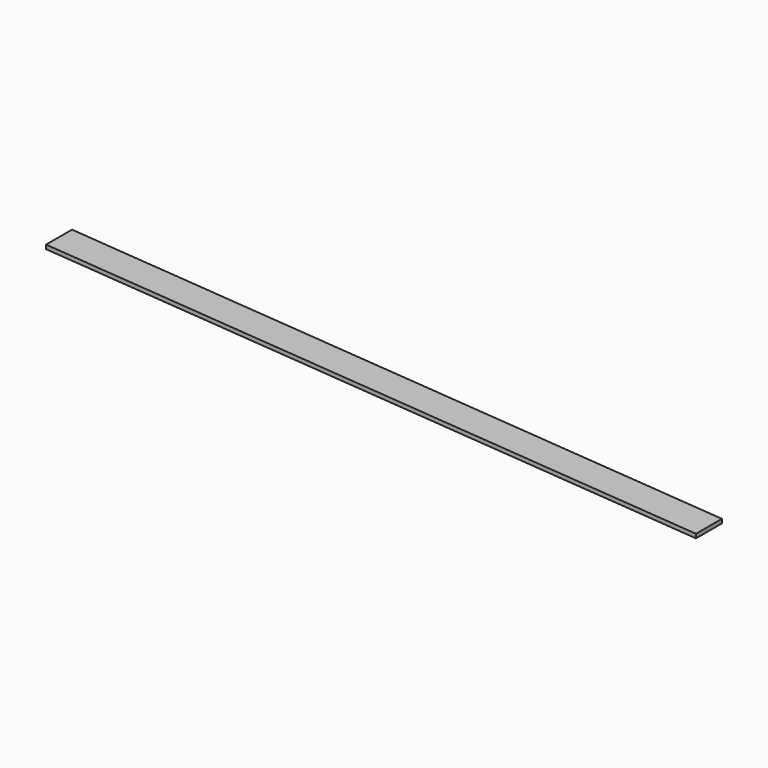
from build123d import *

# Parameters (mm, degrees)
F1_DEPTH = 3.175


with BuildPart() as f1:
    # F0 (on Top) → F1 (new body)
    with BuildSketch(Plane.XY):
        Polygon((-200.6755134484, 25.5390722305), (-200.6755134484, 0.1390722305), (349.2344865516, -50.6609277695), (349.2344865516, -25.2609277695), align=None)
    extrude(amount=F1_DEPTH)


solid = f1.part
